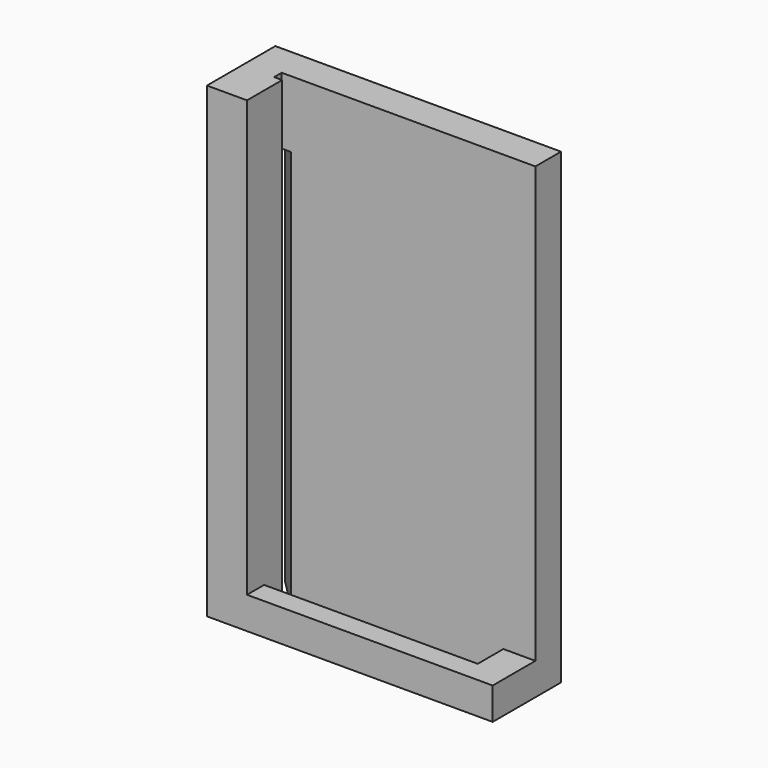
from build123d import *

# Parameters (mm, degrees)
F1_DEPTH = 25
F2_DEPTH = 150
F4_DEPTH = 175
F5_W     = 12
F5_H     = 8
F5_H_2   = 12
F6_DEPTH = 12


with BuildPart() as f1:
    # F0 (on Top) → F1 (new body)
    with BuildSketch(Plane.XY):
        Polygon((-15.4107665035, -11.7272357842), (-11.8752325976, -15.2627696901), (79.5892334965, -15.2627696901), (79.5892334965, -3.2627696901), (-15.4107665035, -3.2627696901), align=None)
        Polygon((-23.8752325976, -3.2627696901), (-15.4107665035, -11.7272357842), (-15.4107665035, -3.2627696901), align=None)
        Polygon((-18.9463004094, -15.2627696901), (-15.4107665035, -15.2627696901), (-27.4107665035, -3.2627696901), (-27.4107665035, -6.7983035961), align=None)
        Polygon((-27.4107665035, -15.2627696901), (-18.9463004094, -15.2627696901), (-27.4107665035, -6.7983035961), align=None)
        Polygon((-15.4107665035, -18.7983035961), (-18.9463004094, -15.2627696901), (-27.4107665035, -15.2627696901), (-27.4107665035, -35.2627696901), (-15.4107665035, -35.2627696901), align=None)
        Polygon((-27.4107665035, -3.2627696901), (-15.4107665035, -15.2627696901), (-15.4107665035, -11.7272357842), (-23.8752325976, -3.2627696901), align=None)
        Polygon((-15.4107665035, -11.7272357842), (-15.4107665035, -15.2627696901), (-11.8752325976, -15.2627696901), align=None)
        Polygon((-15.4107665035, -18.7983035961), (-15.4107665035, -15.2627696901), (-18.9463004094, -15.2627696901), align=None)
    extrude(amount=F1_DEPTH)

    # F0 (on Top) → F2 (join)
    with BuildSketch(Plane.XY):
        Polygon((-15.4107665035, -18.7983035961), (-18.9463004094, -15.2627696901), (-27.4107665035, -15.2627696901), (-27.4107665035, -35.2627696901), (-15.4107665035, -35.2627696901), align=None)
        Polygon((-23.8752325976, -3.2627696901), (-15.4107665035, -11.7272357842), (-15.4107665035, -3.2627696901), align=None)
        Polygon((-15.4107665035, -11.7272357842), (-11.8752325976, -15.2627696901), (79.5892334965, -15.2627696901), (79.5892334965, -3.2627696901), (-15.4107665035, -3.2627696901), align=None)
        Polygon((-27.4107665035, -15.2627696901), (-18.9463004094, -15.2627696901), (-27.4107665035, -6.7983035961), align=None)
    extrude(amount=-F2_DEPTH)

    # F3 (on face) → F4 (join, through all)
    with BuildSketch(Plane(origin=(0, 0, -150), x_dir=(1, 0, 0), z_dir=(0, 0, -1))):
        Polygon((-15.4107665035, 30.7983035961), (-15.4107665035, 18.7983035961), (-12.4107665035, 18.7983035961), (-12.4107665035, 30.7983035961), (-12.4107665035, 35.2627696901), (-15.4107665035, 35.2627696901), align=None)
    extrude(amount=-F4_DEPTH)

    # F5 (on face) → F6 (join)
    with BuildSketch(Plane(origin=(0, 0, -150), x_dir=(1, 0, 0), z_dir=(0, 0, -1))):
        Polygon((-12.4107665035, 35.2627696901), (-12.4107665035, 30.7983035961), (-12.4107665035, 27.2627696901), (67.5892334965, 27.2627696901), (67.5892334965, 35.2627696901), align=None)
        with Locations((73.5892334965, 31.2627696901)):
            Rectangle(F5_W, F5_H)
        with Locations((73.5892334965, 21.2627696901)):
            Rectangle(F5_W, F5_H_2)
        Polygon((79.5892334965, 15.2627696901), (67.5892334965, 15.2627696901), (-11.8752325976, 15.2627696901), (-23.8752325976, 3.2627696901), (79.5892334965, 3.2627696901), align=None)
    extrude(amount=-F6_DEPTH)


solid = f1.part
